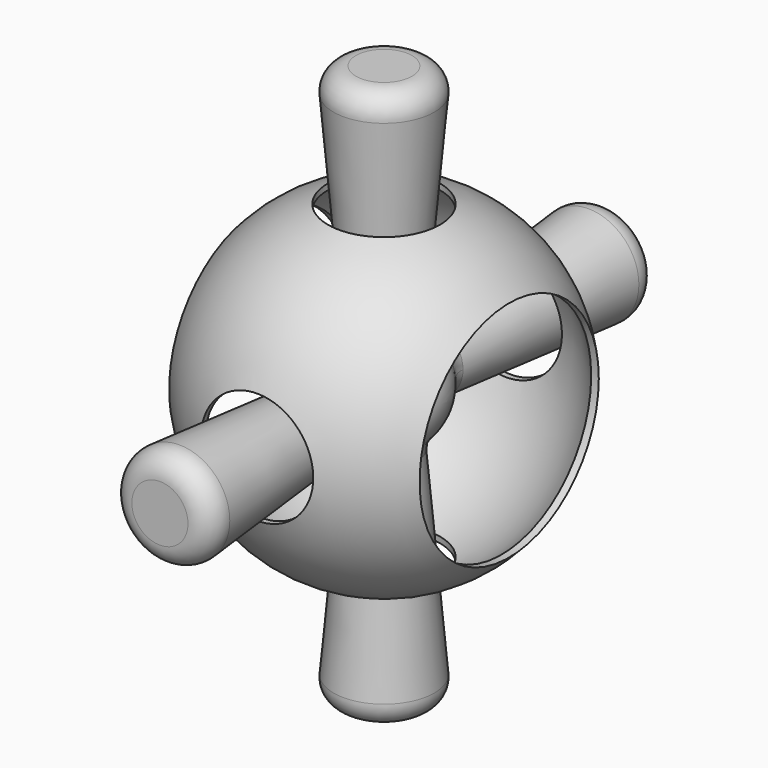
from build123d import *

# Parameters (mm, degrees)
F3_T      = -2.54
F4_DEPTH  = 76.2
F7_R      = 12.7
F8_DEPTH  = 127
F8_TAPER  = -5
F9_R      = 50.8
F10_DEPTH = 76.2
F11_R     = 10.16


# Not quite as in the source:
# - a pattern or mirror of a feature is missing from the dataset's text; its kind, count and spacing are read off the source's solid


with BuildPart() as f1:
    # F0 (on Top) → F1 (revolve)
    with BuildSketch(Plane.XY):
        with BuildLine():
            Line((-76.2, 0), (76.2, 0))
            ThreePointArc((76.2, 0), (0, 76.2), (-76.2, 0))
        make_face()
    revolve(axis=Axis((0, 0, 0), (1, 0, 0)))

    # F3 (hollow: no face is removed)
    offset(amount=F3_T, mode=Mode.SUBTRACT)

    # F2 (on Top) → F4 (cut, symmetric)
    with BuildSketch(Plane.XY):
        with BuildLine():
            Line((-25.4, 0), (25.4, 0))
            ThreePointArc((25.4, 0), (0, 25.4), (-25.4, 0))
        make_face()
        with BuildLine():
            ThreePointArc((-25.4, 0), (0, -25.4), (25.4, 0))
            Line((25.4, 0), (-25.4, 0))
        make_face()
    f4 = extrude(amount=F4_DEPTH, both=True, mode=Mode.SUBTRACT)

    # F4_copies: F4 across plane
    add(f4.mirror(Plane(origin=(0, 0, 0), x_dir=(0, 0.7071067812, 0.7071067812), z_dir=(0, -0.7071067812, 0.7071067812))), mode=Mode.SUBTRACT)

    # F9 (on Right) → F10 (cut, symmetric)
    with BuildSketch(Plane.YZ):
        Circle(F9_R)
    extrude(amount=F10_DEPTH, both=True, mode=Mode.SUBTRACT)


with BuildPart() as f5:
    # F2 (on Top) → F5 (revolve)
    with BuildSketch(Plane.XY):
        with BuildLine():
            Line((-25.4, 0), (25.4, 0))
            ThreePointArc((25.4, 0), (0, 25.4), (-25.4, 0))
        make_face()
    revolve(axis=Axis((0, 0, 0), (-1, 0, 0)))

    # F7 (on Front) → F8 (join, symmetric)
    with BuildSketch(Plane.XZ):
        Circle(F7_R)
    f8 = extrude(amount=F8_DEPTH, both=True, taper=F8_TAPER)

    # F8_copies: F8 across plane
    add(f8.mirror(Plane(origin=(0, 0, 0), x_dir=(0, -0.7071067812, 0.7071067812), z_dir=(0, 0.7071067812, 0.7071067812))))

    # F11
    f11_edges = [f5.edges().sort_by_distance(p)[0] for p in [
        (-23.81106, 127, 0),
        (0, 20.838399, -14.523124),
        (0, 20.838399, 14.523124),
        (-14.523124, 0, -20.838399),
        (-14.523124, 0, 20.838399),
        (-14.523124, -20.838399, 0),
        (-23.81106, 0, -127),
        (-23.81106, 0, 127),
        (-23.81106, -127, 0),
    ]]
    fillet(f11_edges, radius=F11_R)


solid = Compound([f1.part, f5.part])
